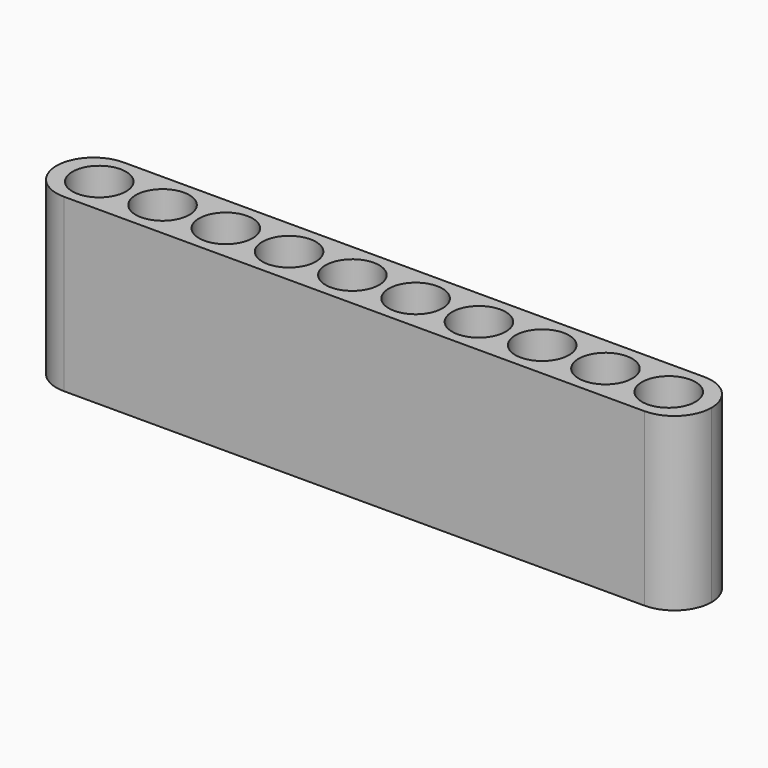
from build123d import *

# Parameters (mm, degrees)
F0_W     = 88
F0_H     = 10
F1_DEPTH = 23
F2_R     = 3.6
F3_DEPTH = 22
F4_R     = 4.99999


# Not quite as in the source:
# - a fillet or chamfer is up to 0.001 mm smaller than in the source, because OpenCascade refuses the exact size


with BuildPart() as f1:
    # F0 (on Top) → F1 (new body)
    with BuildSketch(Plane.XY):
        Rectangle(F0_W, F0_H)
    extrude(amount=F1_DEPTH)

    # F2 (on face) → F3 (cut)
    with BuildSketch(Plane.XY.offset(23)):
        with Locations((-38.25, 0)):
            Circle(F2_R)
        with Locations((-29.75, 0)):
            Circle(F2_R)
        with Locations((-21.25, 0)):
            Circle(F2_R)
        with Locations((-12.75, 0)):
            Circle(F2_R)
        with Locations((-4.25, 0)):
            Circle(F2_R)
        with Locations((4.25, 0)):
            Circle(F2_R)
        with Locations((12.75, 0)):
            Circle(F2_R)
        with Locations((21.25, 0)):
            Circle(F2_R)
        with Locations((29.75, 0)):
            Circle(F2_R)
        with Locations((38.25, 0)):
            Circle(F2_R)
    extrude(amount=-F3_DEPTH, mode=Mode.SUBTRACT)

    # F4 (radius 5 in the source; OpenCascade refuses exactly that, so slightly less here)
    f4_edges = [f1.edges().sort_by_distance(p)[0] for p in [
        (44, 5, 11.5),
        (44, -5, 11.5),
        (-44, -5, 11.5),
        (-44, 5, 11.5),
    ]]
    fillet(f4_edges, radius=F4_R)


solid = f1.part
